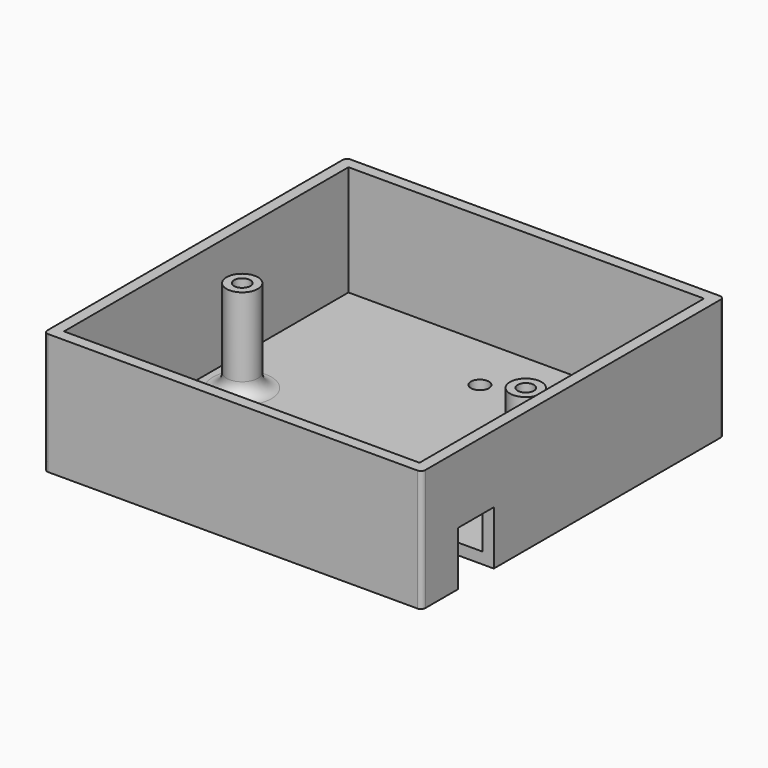
from build123d import *

# Parameters (mm, degrees)
F0_W      = 84
F0_H      = 84
F1_DEPTH  = 27
F2_T      = -2.5
F3_DEPTH  = 2
F4_W      = 65
F4_H      = 14
F5_DEPTH  = 25
F6_W      = 10
F6_H      = 10
F7_DEPTH  = 21.8
F4_R      = 2
F8_DEPTH  = 25
F9_DEPTH  = 2
F10_R     = 3.5
F10_R_2   = 1.8
F11_DEPTH = 21
F12_DEPTH = 10
F13_R     = 1
F14_DEPTH = 2
F15_R     = 3


# Not quite as in the source:
# - a feature names something its author has since deleted; it is built from what else it names


with BuildPart() as f1:
    # F0 (on Top) → F1 (new body)
    with BuildSketch(Plane.XY):
        Rectangle(F0_W, F0_H)
    extrude(amount=F1_DEPTH)

    # F2
    f2_openings = [f1.faces().sort_by_distance(p)[0] for p in [
        (0, 0, 27),
    ]]
    offset(amount=F2_T, openings=f2_openings)

    # F3 (cut): a face of the model
    f3_faces = [f1.faces().sort_by_distance(p)[0] for p in [
        (0, 0, 2.5),
    ]]
    extrude(f3_faces, amount=F3_DEPTH, mode=Mode.SUBTRACT)

    # F4 (on face) → F5 (cut)
    with BuildSketch(Plane.XY.offset(2.5)):
        with Locations((0, -27)):
            Rectangle(F4_W, F4_H)
    extrude(amount=-F5_DEPTH, mode=Mode.SUBTRACT)

    # F6 (on face) → F7 (cut)
    with BuildSketch(Plane.YZ.offset(42)):
        with Locations((-27, 5)):
            Rectangle(F6_W, F6_H)
    extrude(amount=-F7_DEPTH, mode=Mode.SUBTRACT)

    # F4 (on face) → F8 (cut)
    with BuildSketch(Plane.XY.offset(2.5)):
        with Locations((0, 26.6423244029)):
            Circle(F4_R)
        with Locations((0, -10.8067262918)):
            Circle(F4_R)
    extrude(amount=-F8_DEPTH, mode=Mode.SUBTRACT)

    # F9 (cut): faces of the model
    f9_faces = [f1.faces().sort_by_distance(p)[0] for p in [
        (0, 40.8120606076, 27),
        (-0.4812956241, 5.0155977429, 2.5),
    ]]
    extrude(f9_faces, amount=-F9_DEPTH, mode=Mode.SUBTRACT)

    # F10 (on Top) → F11 (join)
    with BuildSketch(Plane.XY):
        with Locations((-31.5, 0)):
            Circle(F10_R)
        with Locations((-31.5, 0)):
            Circle(F10_R_2, mode=Mode.SUBTRACT)
        with Locations((31.5, 0)):
            Circle(F10_R)
        with Locations((31.5, 0)):
            Circle(F10_R_2, mode=Mode.SUBTRACT)
    extrude(amount=F11_DEPTH)

    # F10 (on Top) → F12 (join)
    with BuildSketch(Plane.XY):
        with Locations((-31.5, 0)):
            Circle(F10_R_2)
        with Locations((31.5, 0)):
            Circle(F10_R_2)
    extrude(amount=F12_DEPTH)

    # F13
    f13_edges = [f1.edges().sort_by_distance(p)[0] for p in [
        (-42, 42, 12.5),
        (42, 42, 12.5),
        (42, -42, 12.5),
        (-42, -42, 12.5),
    ]]
    fillet(f13_edges, radius=F13_R)

    # F14 (add): a face of the model
    f14_faces = [f1.faces().sort_by_distance(p)[0] for p in [
        (-0.5873435355, 4.470699491, 0),
    ]]
    extrude(f14_faces, amount=F14_DEPTH)

    # F15
    f15_edges = [f1.edges().sort_by_distance(p)[0] for p in [
        (-35, 0, 0.5),
        (28, 0, 0.5),
    ]]
    fillet(f15_edges, radius=F15_R)


solid = f1.part
